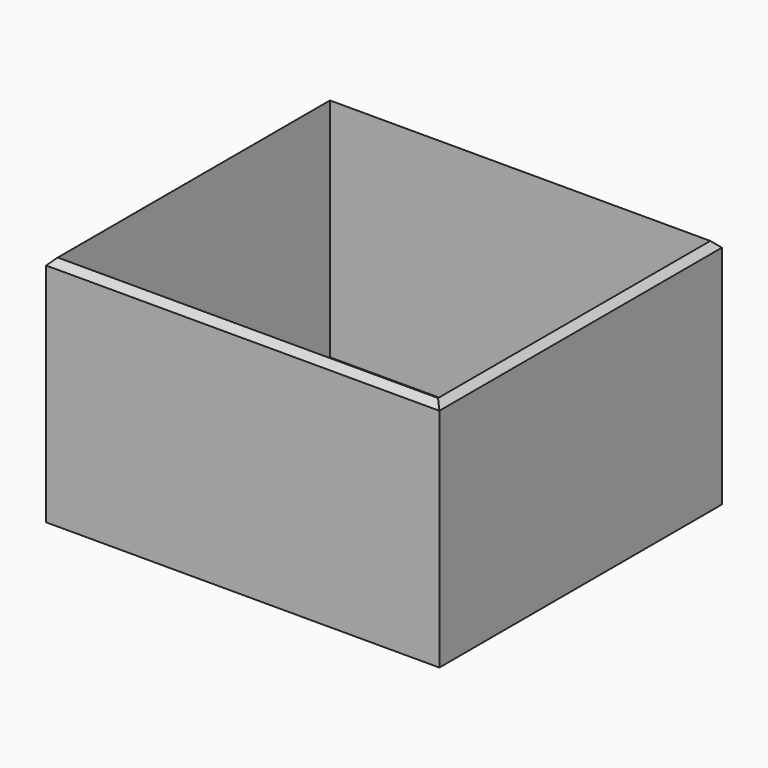
from build123d import *

# Parameters (mm, degrees)
F0_W        = 77.315364033
F0_H        = 69.4387331605
F1_DEPTH    = 50.8
F2_T        = -1.27
F3_T1_DEPTH = 109.9757379802
F3_T3_DEPTH = 102.0991071077


# Not quite as in the source:
# - a fillet or chamfer that OpenCascade refuses, or shapes differently, is made with other operations: its cross-section is extruded or revolved along the edge and cut away or added
# - the program builds the solid bodies; features that only make, move or delete a surface that nothing else refers to are left out


with BuildPart() as f1:
    # F0 (on Top) → F1 (new body)
    with BuildSketch(Plane.XY):
        with Locations((-0.1036394387, -4.8710741103)):
            Rectangle(F0_W, F0_H)
    extrude(amount=F1_DEPTH)

    # F2
    f2_openings = [f1.faces().sort_by_distance(p)[0] for p in [
        (-0.103639, -4.871074, 50.8),
    ]]
    offset(amount=F2_T, openings=f2_openings)

    # F3: chamfer of 6.35 on 4 edges, made by hand

    # F3_s2 → F3_t1 (cut)
    with BuildSketch(Plane.YZ.offset(-55.0915084288)):
        Polygon((-39.5904406905, 44.45), (-33.2404406905, 50.8), (-39.5904406905, 50.8), align=None)
        Polygon((29.84829247, 44.45), (23.49829247, 50.8), (29.84829247, 50.8), align=None)
    extrude(amount=F3_T1_DEPTH, mode=Mode.SUBTRACT)

    # F3_s4 → F3_t3 (cut)
    with BuildSketch(Plane.XZ.offset(-46.1784794436)):
        Polygon((-38.7613214552, 44.45), (-32.4113214552, 50.8), (-38.7613214552, 50.8), align=None)
        Polygon((38.5540425777, 44.45), (32.2040425777, 50.8), (38.5540425777, 50.8), align=None)
    extrude(amount=F3_T3_DEPTH, mode=Mode.SUBTRACT)


solid = f1.part
